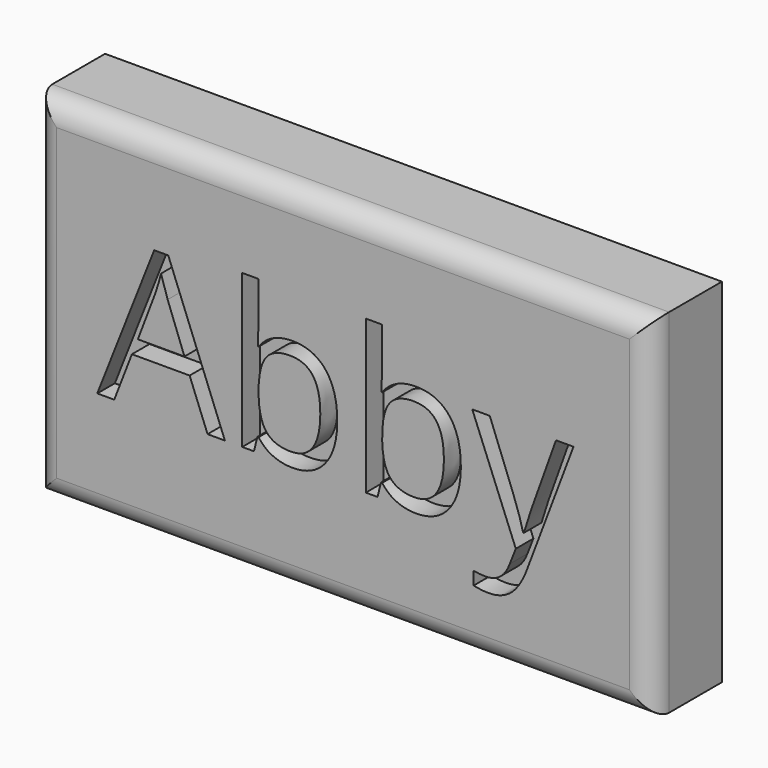
from build123d import *

# Parameters (mm, degrees)
F0_W         = 177.9485046864
F0_H         = 101.7419733107
F1_DEPTH     = 25.4
F2_R         = 6.35
F3_TEXT_SIZE = 58.1790143365
F4_DEPTH     = 6.35


# Not quite as in the source:
# - Text() gives the source's letters only with a copy of the font that has no kerning and outlines rounded to 1/6400 em; it was checked with that copy


with BuildPart() as f1:
    # F0 (on Front) → F1 (new body)
    with BuildSketch(Plane.XZ):
        with Locations((12.3964995146, 16.9717352837)):
            Rectangle(F0_W, F0_H)
    extrude(amount=F1_DEPTH)

    # F2
    f2_edges = [f1.edges().sort_by_distance(p)[0] for p in [
        (12.3965, -25.4, 67.842722),
        (-76.577753, -25.4, 16.971735),
        (12.3965, -25.4, -33.899251),
        (101.370752, -25.4, 16.971735),
    ]]
    fillet(f2_edges, radius=F2_R)

    # F3 (on face) → F4 (cut)
    with BuildSketch(Plane.XZ.offset(25.4)):
        with Locations((-58.5114676505, -2.2163442336)):
            Text('Abby', F3_TEXT_SIZE, font='Open Sans', text_align=(TextAlign.LEFT, TextAlign.BOTTOM))
    extrude(amount=-F4_DEPTH, mode=Mode.SUBTRACT)


solid = f1.part
